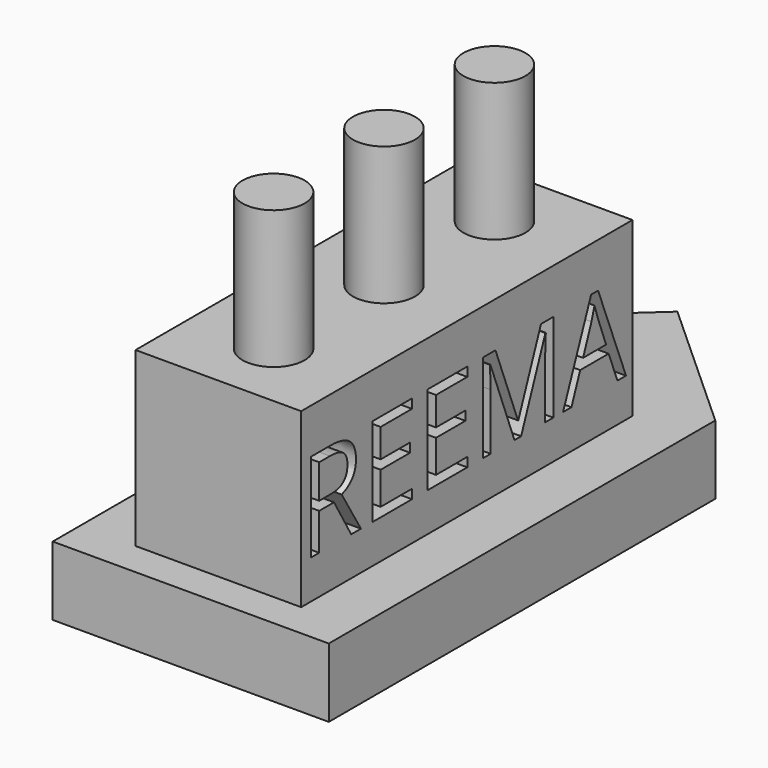
from build123d import *

# Parameters (mm, degrees)
F1_DEPTH     = 10
F2_W         = 24
F2_H         = 60
F3_DEPTH     = 25
F4_R         = 4.5
F5_DEPTH     = 20
F6_TEXT_SIZE = 24.3929874462
F8_DEPTH     = 5
F7_TEXT_SIZE = 18.0137918094
F9_DEPTH     = 5


# Not quite as in the source:
# - Text() gives the source's letters only with a copy of the font that has no kerning and outlines rounded to 1/6400 em; it was checked with that copy


with BuildPart() as f1:
    # F0 (on Top) → F1 (new body)
    with BuildSketch(Plane.XY):
        Polygon((-20, 35), (-20, -35), (20, -35), (20, 35), (0, 53.1383571472), align=None)
    extrude(amount=F1_DEPTH)

    # F2 (on face) → F3 (join)
    with BuildSketch(Plane.XY.offset(10)):
        Rectangle(F2_W, F2_H)
    extrude(amount=F3_DEPTH)

    # F4 (on face) → F5 (join)
    with BuildSketch(Plane.XY.offset(35)):
        Circle(F4_R)
        with Locations((0, 20)):
            Circle(F4_R)
        with Locations((0, -20)):
            Circle(F4_R)
    extrude(amount=F5_DEPTH)

    # F6 (on face) → F8 (cut)
    with BuildSketch(Plane(origin=(-12, 0, 0), x_dir=(0, -1, 0), z_dir=(-1, 0, 0))):
        with Locations((-30, 12.8889391199)):
            Text('M.sh', F6_TEXT_SIZE, font='Open Sans', text_align=(TextAlign.LEFT, TextAlign.BOTTOM))
    extrude(amount=-F8_DEPTH, mode=Mode.SUBTRACT)

    # F7 (on face) → F9 (cut)
    with BuildSketch(Plane.YZ.offset(12)):
        with Locations((-30, 15.6103603515)):
            Text('REEMA', F7_TEXT_SIZE, font='Open Sans', text_align=(TextAlign.LEFT, TextAlign.BOTTOM))
    extrude(amount=-F9_DEPTH, mode=Mode.SUBTRACT)


solid = f1.part
